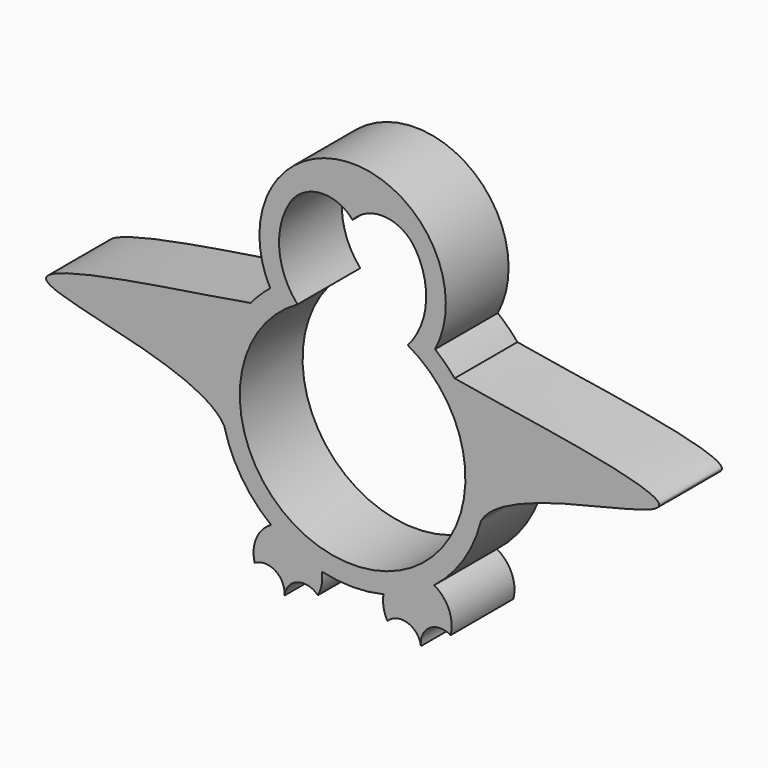
from build123d import *

# Parameters (mm, degrees)
F1_DEPTH = 25.4


# Not quite as in the source:
# - a feature names something its author has since deleted; it is built from what else it names


with BuildPart() as f1:
    # F0 (on Front) → F1 (new body)
    with BuildSketch(Plane.XZ):
        with BuildLine():
            ThreePointArc((33.018049972, 14.6313424898), (30.0088601414, 17.9049378249), (26.6767187304, 20.8491666667))
            ThreePointArc((26.6767187304, 20.8491666667), (0, 65.0875), (-26.6767187304, 20.8491666667))
            ThreePointArc((-26.6767187304, 20.8491666667), (-30.0088601414, 17.9049378249), (-33.018049972, 14.6313424898))
            ThreePointArc((-33.018049972, 14.6313424898), (-41.8158398527, -3.2856787995), (-41.5452899235, -23.2443250813))
            ThreePointArc((-41.5452899235, -23.2443250813), (-35.8973631324, -36.1216401303), (-26.3860544261, -46.4782480018))
            ThreePointArc((-26.3860544261, -46.4782480018), (-18.6113486842, -51.3110295952), (-9.9877042304, -54.3826063299))
            ThreePointArc((-9.9877042304, -54.3826063299), (0, -55.5625), (9.9877042304, -54.3826063299))
            ThreePointArc((9.9877042304, -54.3826063299), (18.6113486842, -51.3110295952), (26.3860544261, -46.4782480018))
            ThreePointArc((26.3860544261, -46.4782480018), (35.8973631324, -36.1216401303), (41.5452899235, -23.2443250813))
            ThreePointArc((41.5452899235, -23.2443250813), (41.8158398527, -3.2856787995), (33.018049972, 14.6313424898))
        make_face()
        with BuildLine():
            ThreePointArc((20.4107142857, 47.190312821), (23.7132340956, 32.7529767549), (17.8428848253, 19.1558333333))
            ThreePointArc((17.8428848253, 19.1558333333), (0, -49.2125), (-17.8428848253, 19.1558333333))
            ThreePointArc((-17.8428848253, 19.1558333333), (-23.7132340956, 32.7529767549), (-20.4107142857, 47.190312821))
            ThreePointArc((-20.4107142857, 47.190312821), (-10.6767956636, 53.2964751512), (0, 49.0490730624))
            ThreePointArc((0, 49.0490730624), (10.6767956636, 53.2964751512), (20.4107142857, 47.190312821))
        make_face(mode=Mode.SUBTRACT)
        with BuildLine():
            ThreePointArc((31.7028005699, -58.996710055), (31.1832359324, -51.8291005513), (26.3860544261, -46.4782480018))
            ThreePointArc((26.3860544261, -46.4782480018), (18.6113486842, -51.3110295952), (9.9877042304, -54.3826063299))
            ThreePointArc((9.9877042304, -54.3826063299), (10.009677281, -58.0934630853), (11.2522370234, -61.5901738197))
            ThreePointArc((11.2522370234, -61.5901738197), (17.8174676094, -59.9971626047), (22.102310986, -65.220193776))
            ThreePointArc((22.102310986, -65.220193776), (24.9477521066, -59.0929266684), (31.7028005699, -58.996710055))
        make_face()
        with BuildLine():
            ThreePointArc((-9.9877042304, -54.3826063299), (-18.6113486842, -51.3110295952), (-26.3860544261, -46.4782480018))
            ThreePointArc((-26.3860544261, -46.4782480018), (-31.1832359324, -51.8291005513), (-31.7028005699, -58.996710055))
            ThreePointArc((-31.7028005699, -58.996710055), (-24.9477521066, -59.0929266684), (-22.102310986, -65.220193776))
            ThreePointArc((-22.102310986, -65.220193776), (-17.8174676094, -59.9971626047), (-11.2522370234, -61.5901738197))
            ThreePointArc((-11.2522370234, -61.5901738197), (-10.009677281, -58.0934630853), (-9.9877042304, -54.3826063299))
        make_face()
        with BuildLine():
            add(Edge.make_bspline(
                [(33.018049972, 14.6313424898), (46.9965733011, 11.8619536122), (150.360470689, -0.7954577234), (49.0987253283, -9.3555527531), (41.5452899235, -23.2443250813)],
                knots=[0, 0, 0, 0, 0.5108094749, 1, 1, 1, 1], degree=3))
            ThreePointArc((33.018049972, 14.6313424898), (41.8158398527, -3.2856787995), (41.5452899235, -23.2443250813))
        make_face()
        with BuildLine():
            ThreePointArc((-41.5452899235, -23.2443250813), (-41.8158398527, -3.2856787995), (-33.018049972, 14.6313424898))
            add(Edge.make_bspline(
                [(-33.018049972, 14.6313424898), (-46.9965733011, 11.8619536122), (-150.360470689, -0.7954577234), (-49.0987253283, -9.3555527531), (-41.5452899235, -23.2443250813)],
                knots=[0, 0, 0, 0, 0.5108094749, 1, 1, 1, 1], degree=3))
        make_face()
    extrude(amount=F1_DEPTH)


solid = f1.part
